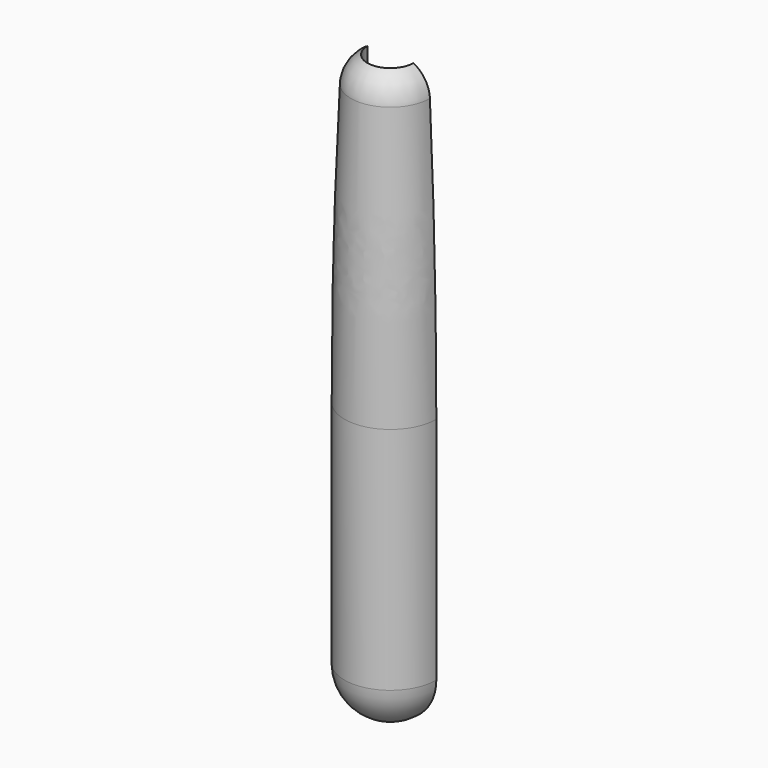
from build123d import *

# Parameters (mm, degrees)
F1_ANGLE    = 180
F2_T2_ANGLE = 359.64


# Not quite as in the source:
# - a fillet or chamfer that OpenCascade refuses, or shapes differently, is made with other operations: its cross-section is extruded or revolved along the edge and cut away or added


with BuildPart() as f1:
    # F0 (on Front) → F1 (revolve)
    with BuildSketch(Plane.XZ):
        with BuildLine():
            ThreePointArc((-2, 2.2360679775), (-2.7386127875, 1.2247448714), (-3, 0))
            ThreePointArc((-3, 0), (-2.1213203436, -2.1213203436), (0, -3))
            Line((0, -3), (0, 0))
            Line((0, 0), (-2, 0))
            Line((-2, 0), (-2, 2.2360679775))
        make_face()
        with BuildLine():
            Line((-3, 15), (-3, 0))
            ThreePointArc((-3, 0), (-2.7386127875, 1.2247448714), (-2, 2.2360679775))
            Line((-2, 2.2360679775), (-2, 15))
            Line((-2, 15), (-1.5, 15))
            Line((-1.5, 15), (-1.5, 35))
            Line((-1.5, 35), (-2.5, 35))
            ThreePointArc((-2.5, 35), (-2.8749804749, 25.0031245119), (-3, 15))
        make_face()
    revolve(axis=Axis((0, 0, 7.5), (0, 0, 1)), revolution_arc=F1_ANGLE)

    # F2: fillet of radius 2 on 1 edges, made by hand

    # F2_s1 → F2_t2 (revolve, cut)
    with BuildSketch(Plane(origin=(0, 0, 0), x_dir=(0, 0, 1), z_dir=(0.9999950652, 0.0031415875, 0))):
        with BuildLine():
            ThreePointArc((35, -1.5), (34.3021016304, -2.2665733355), (33.3141893252, -2.5807804176))
            Line((33.3141893252, -2.5807804176), (33.3160196002, -2.6207385218))
            ThreePointArc((33.3160196002, -2.6207385218), (34.1590517584, -2.5812329417), (35.0019987508, -2.5399500312))
            Line((35.0019987508, -2.5399500312), (35.04, -2.5))
            ThreePointArc((35.04, -2.5), (35.04, -2), (35.0355464885, -1.5183424959))
            Line((35.0355464885, -1.5183424959), (35, -1.5))
        make_face()
    revolve(axis=Axis((0, 0, 35), (0, 0, 1)), revolution_arc=F2_T2_ANGLE, mode=Mode.SUBTRACT)


solid = f1.part
